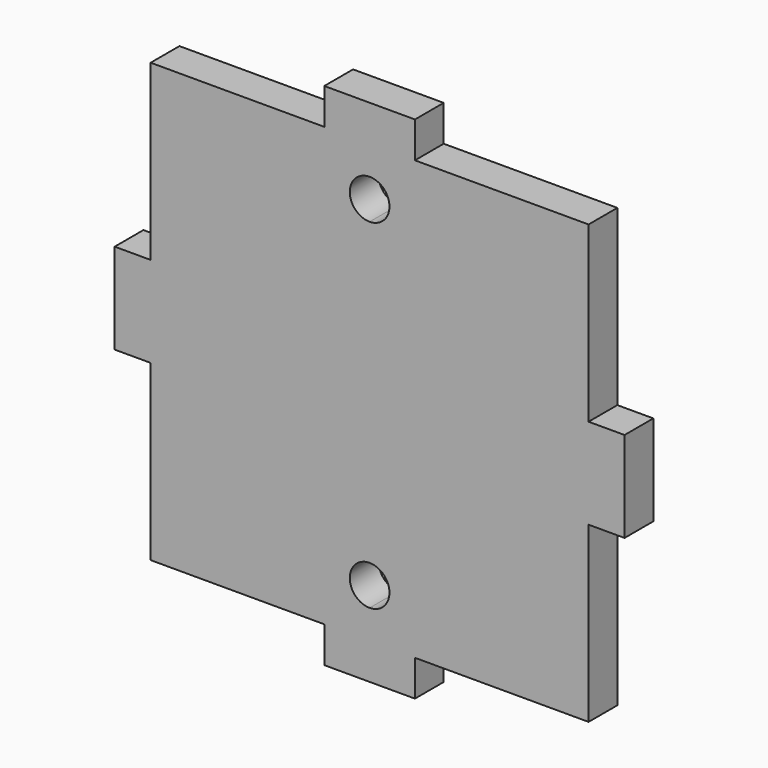
from build123d import *

# Parameters (mm, degrees)
F1_DEPTH = 3.175


# Not quite as in the source:
# - a length typed as a fraction of an inch, garbled in the dataset ("3 / 203.2 mm" for 3/8 in), is restored


with BuildPart() as f1:
    # F0 (on Front) → F1 (new body)
    with BuildSketch(Plane.XZ):
        Polygon((-22.5, -4), (-19.325, -4), (-19.325, -19.325), (-4, -19.325), (-4, -22.5), (0, -22.5), (0, -18), (-18, -18), (-18, 0), (-22.5, 0), align=None)
        Polygon((-22.5, 4), (-22.5, 0), (-18, 0), (-18, 18), (0, 18), (0, 22.5), (-4, 22.5), (-4, 19.325), (-19.325, 19.325), (-19.325, 4), align=None)
        Polygon((0, -18), (0, -22.5), (4, -22.5), (4, -19.325), (19.325, -19.325), (19.325, -4), (22.5, -4), (22.5, 0), (18, 0), (18, -18), align=None)
        Polygon((18, 18), (18, 0), (22.5, 0), (22.5, 4), (19.325, 4), (19.325, 19.325), (4, 19.325), (4, 22.5), (0, 22.5), (0, 18), align=None)
        with BuildLine():
            Line((-18, 18), (-18, 0))
            Line((-18, 0), (0, 0))
            Line((0, 0), (0, 13.25))
            ThreePointArc((0, 13.25), (-1.75, 15), (0, 16.75))
            Line((0, 16.75), (0, 18))
            Line((0, 18), (-18, 18))
        make_face()
        with BuildLine():
            Line((0, 13.25), (0, 0))
            Line((0, 0), (18, 0))
            Line((18, 0), (18, 18))
            Line((18, 18), (0, 18))
            Line((0, 18), (0, 16.75))
            ThreePointArc((0, 16.75), (1.2374368671, 16.2374368671), (1.75, 15))
            ThreePointArc((1.75, 15), (1.2374368671, 13.7625631329), (0, 13.25))
        make_face()
        with BuildLine():
            Line((18, 0), (0, 0))
            Line((0, 0), (0, -13.25))
            ThreePointArc((0, -13.25), (1.2374368671, -13.7625631329), (1.75, -15))
            ThreePointArc((1.75, -15), (1.2374368671, -16.2374368671), (0, -16.75))
            Line((0, -16.75), (0, -18))
            Line((0, -18), (18, -18))
            Line((18, -18), (18, 0))
        make_face()
        with BuildLine():
            Line((0, 0), (-18, 0))
            Line((-18, 0), (-18, -18))
            Line((-18, -18), (0, -18))
            Line((0, -18), (0, -16.75))
            ThreePointArc((0, -16.75), (-1.75, -15), (0, -13.25))
            Line((0, -13.25), (0, 0))
        make_face()
    extrude(amount=F1_DEPTH)


solid = f1.part
